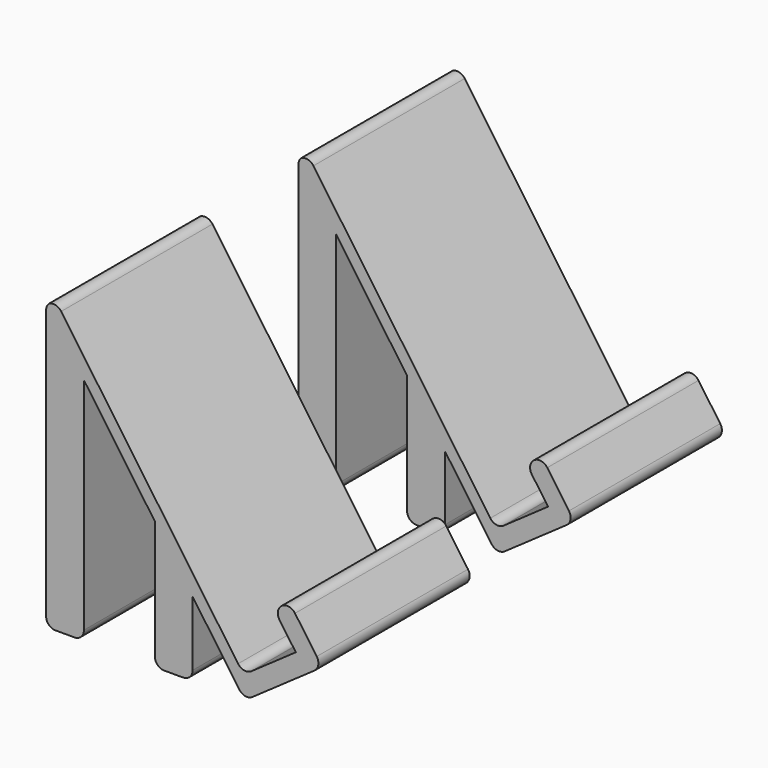
from build123d import *

# Parameters (mm, degrees)
F1_DEPTH    = 101.6
F3_DEPTH    = 6.35
F5_DEPTH    = 44.45
F6_W        = 10.16
F6_H        = 101.6
F7_DEPTH    = 20.32
F8_T1_DEPTH = 101.6
F8_T3_DEPTH = 127
F8_T5_DEPTH = 114.822403084


# Not quite as in the source:
# - a fillet or chamfer that OpenCascade refuses, or shapes differently, is made with other operations: its cross-section is extruded or revolved along the edge and cut away or added


with BuildPart() as f1:
    # F0 (on Front) → F1 (new body)
    with BuildSketch(Plane.XZ):
        Polygon((57.3137016242, -18.4824153282), (36.9937016242, 10.5375521688), (36.9937016242, -58.4300412773), (57.3137016242, -58.4300412773), align=None)
    extrude(amount=F1_DEPTH)



with BuildPart() as f1b:
    # F0 (on Front) → F1, piece 2 (new body)
    with BuildSketch(Plane.XZ):
        Polygon((-1.1062983758, 64.9499912257), (-21.4262983758, 93.9699587227), (-21.4262983758, -58.4300412773), (-1.1062983758, -58.4300412773), align=None)
    extrude(amount=F1_DEPTH)


with BuildPart() as f1_1:
    add(f1.part)

    add(f1b.part)  # F3 merges F1b
    # F2 (on face) → F3 (join)
    with BuildSketch(Plane(origin=(29.774176385, 0, 20.8481027487), x_dir=(0, 1, 0), z_dir=(0.8191520443, 0, 0.5735764364))):
        Polygon((-101.6, 89.265303656), (-101.6, -96.780755544), (0, -96.780755544), (0, 38.465303656), (0, 89.265303656), align=None)
    extrude(amount=F3_DEPTH)

    # F4 (on face) → F5 (join)
    with BuildSketch(Plane(origin=(34.9757918662, 0, 24.4903131196), x_dir=(0, 1, 0), z_dir=(0.8191520443, 0, 0.5735764364))):
        Polygon((-101.6, -86.620755544), (-101.6, -96.780755544), (0, -96.780755544), (0, -86.620755544), (-12.7, -86.620755544), (-88.9, -86.620755544), align=None)
    extrude(amount=F5_DEPTH)

    # F6 (on face) → F7 (join)
    with BuildSketch(Plane(origin=(49.6836242789, 0, -70.9555689817), x_dir=(0.8191520443, 0, 0.5735764364), z_dir=(-0.5735764364, 0, 0.8191520443))):
        with Locations((82.0675579321, -50.8)):
            Rectangle(F6_W, F6_H)
    extrude(amount=F7_DEPTH)

    # F8: fillet of radius 5.08 on 11 edges, made by hand

    # F8_s2 → F8_t1 (join)
    with BuildSketch(Plane.XZ):
        with BuildLine():
            ThreePointArc((81.7456478485, -42.3039634771), (85.0248074909, -44.3930185658), (88.8207085301, -43.5514875655))
            Line((88.8207085301, -43.5514875655), (84.6594161452, -46.4652558621))
            Line((84.6594161452, -46.4652558621), (81.7456478485, -42.3039634771))
        make_face()
    extrude(amount=F8_T1_DEPTH)

    # F8_s4 → F8_t3 (cut)
    with BuildSketch(Plane.XZ.offset(-12.7)):
        with BuildLine():
            ThreePointArc((112.3294196238, -8.4859061114), (109.0502599814, -6.3968510227), (105.2543589422, -7.238382023))
            Line((105.2543589422, -7.238382023), (109.4156513272, -4.3246137264))
            Line((109.4156513272, -4.3246137264), (112.3294196238, -8.4859061114))
        make_face()
        with BuildLine():
            ThreePointArc((122.7369687221, -32.206136333), (124.8260238108, -28.9269766905), (123.9844928105, -25.1310756513))
            Line((123.9844928105, -25.1310756513), (126.8982611071, -29.2923680363))
            Line((126.8982611071, -29.2923680363), (122.7369687221, -32.206136333))
        make_face()
        with BuildLine():
            ThreePointArc((105.2543589422, -7.238382023), (103.1653038535, -10.5175416655), (104.0068348538, -14.3134427047))
            Line((104.0068348538, -14.3134427047), (101.0930665572, -10.1521503197))
            Line((101.0930665572, -10.1521503197), (105.2543589422, -7.238382023))
        make_face()
        with BuildLine():
            ThreePointArc((-13.3109145979, 93.4508767085), (-16.5900742404, 95.5399317971), (-20.3859752796, 94.6984007968))
            Line((-20.3859752796, 94.6984007968), (-16.2246828946, 97.6121690935))
            Line((-16.2246828946, 97.6121690935), (-13.3109145979, 93.4508767085))
        make_face()
        with BuildLine():
            ThreePointArc((82.3715689606, -54.2687586179), (85.650728603, -56.3578137066), (89.4466296422, -55.5162827063))
            Line((89.4466296422, -55.5162827063), (85.2853372573, -58.4300510029))
            Line((85.2853372573, -58.4300510029), (82.3715689606, -54.2687586179))
        make_face()
        with BuildLine():
            ThreePointArc((-16.3462983758, -58.4300412773), (-19.9384008243, -56.9421437258), (-21.4262983758, -53.3500412773))
            Line((-21.4262983758, -53.3500412773), (-21.4262983758, -58.4300412773))
            Line((-21.4262983758, -58.4300412773), (-16.3462983758, -58.4300412773))
        make_face()
        with BuildLine():
            ThreePointArc((-1.1062983758, -53.3500412773), (-2.5941959274, -56.9421437258), (-6.1862983758, -58.4300412773))
            Line((-6.1862983758, -58.4300412773), (-1.1062983758, -58.4300412773))
            Line((-1.1062983758, -58.4300412773), (-1.1062983758, -53.3500412773))
        make_face()
        with BuildLine():
            ThreePointArc((36.9937016242, -53.3500412773), (38.4815991757, -56.9421437258), (42.0737016242, -58.4300412773))
            Line((42.0737016242, -58.4300412773), (36.9937016242, -58.4300412773))
            Line((36.9937016242, -58.4300412773), (36.9937016242, -53.3500412773))
        make_face()
        with BuildLine():
            ThreePointArc((52.2337016242, -58.4300412773), (55.8258040726, -56.9421437258), (57.3137016242, -53.3500412773))
            Line((57.3137016242, -53.3500412773), (57.3137016242, -58.4300412773))
            Line((57.3137016242, -58.4300412773), (52.2337016242, -58.4300412773))
        make_face()
    extrude(amount=F8_T3_DEPTH, mode=Mode.SUBTRACT)

    # F8_s6 → F8_t5 (cut)
    with BuildSketch(Plane.XZ.offset(-6.611201542)):
        with BuildLine():
            ThreePointArc((-21.4262983758, 91.3254781059), (-20.8523134084, 93.6711610611), (-19.2600666725, 95.4867704908))
            Line((-19.2600666725, 95.4867704908), (-21.4262983758, 93.9699587227))
            Line((-21.4262983758, 93.9699587227), (-21.4262983758, 91.3254781059))
        make_face()
    extrude(amount=F8_T5_DEPTH, mode=Mode.SUBTRACT)


with BuildPart() as f9_1:
    # F9: copy of F1
    add(f1_1.part.moved(Location((0, 169.418, 0))))


solid = Compound([f1_1.part, f9_1.part])
